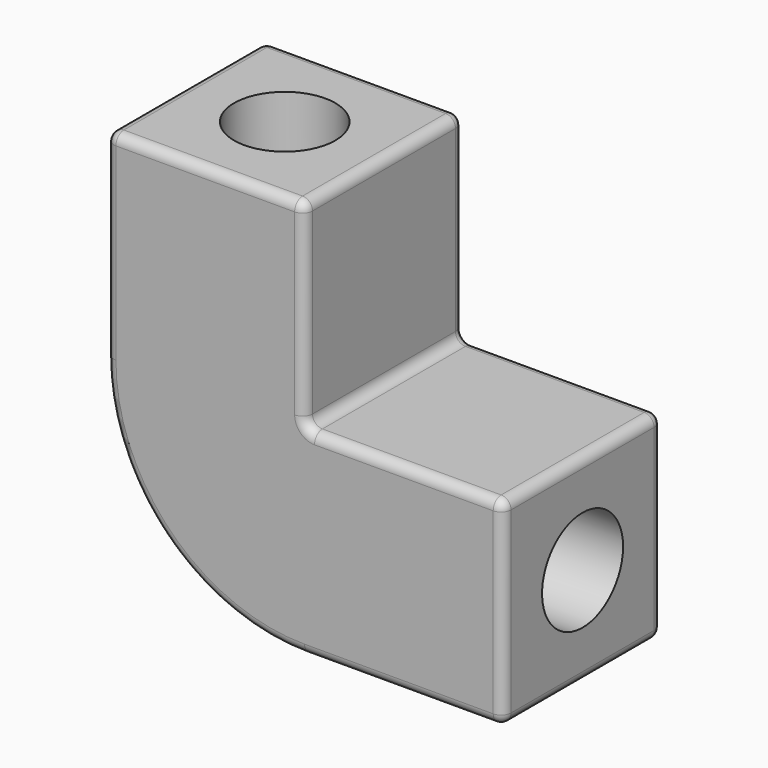
from build123d import *

# Parameters (mm, degrees)
F0_W     = 20
F0_H     = 20
F1_DEPTH = 20
F2_R     = 1
F3_R     = 5.1
F4_DEPTH = 20
F5_R     = 5.1
F6_DEPTH = 20


with BuildPart() as f1:
    # F0 (on Front) → F1 (new body)
    with BuildSketch(Plane.XZ):
        with Locations((-10, 30)):
            Rectangle(F0_W, F0_H)
        with Locations((10, 10)):
            Rectangle(F0_W, F0_H)
        Polygon((-20, 20), (0, 0), (0, 20), align=None)
        with BuildLine():
            ThreePointArc((-20, 20), (-14.1421356237, 5.8578643763), (0, 0))
            Line((0, 0), (-20, 20))
        make_face()
    extrude(amount=F1_DEPTH)

    # F2
    f2_edges = [f1.edges().sort_by_distance(p)[0] for p in [
        (0, -20, 30),
        (0, -10, 40),
        (-10, -20, 40),
        (-20, -10, 40),
        (10, -20, 20),
        (10, 0, 20),
        (20, -10, 20),
        (20, -20, 10),
        (20, 0, 10),
        (20, -10, 0),
        (10, -20, 0),
        (-20, -20, 30),
        (0, 0, 30),
        (-10, 0, 40),
        (-20, 0, 30),
        (10, 0, 0),
        (-14.142136, -20, 5.857864),
        (0, -10, 20),
    ]]
    fillet(f2_edges, radius=F2_R)

    # F3 (on face) → F4 (cut)
    with BuildSketch(Plane.XY.offset(40)):
        with Locations((-10, -10)):
            Circle(F3_R)
    extrude(amount=-F4_DEPTH, mode=Mode.SUBTRACT)

    # F5 (on face) → F6 (cut)
    with BuildSketch(Plane.YZ.offset(20)):
        with Locations((-10, 10)):
            Circle(F5_R)
    extrude(amount=-F6_DEPTH, mode=Mode.SUBTRACT)


solid = f1.part
